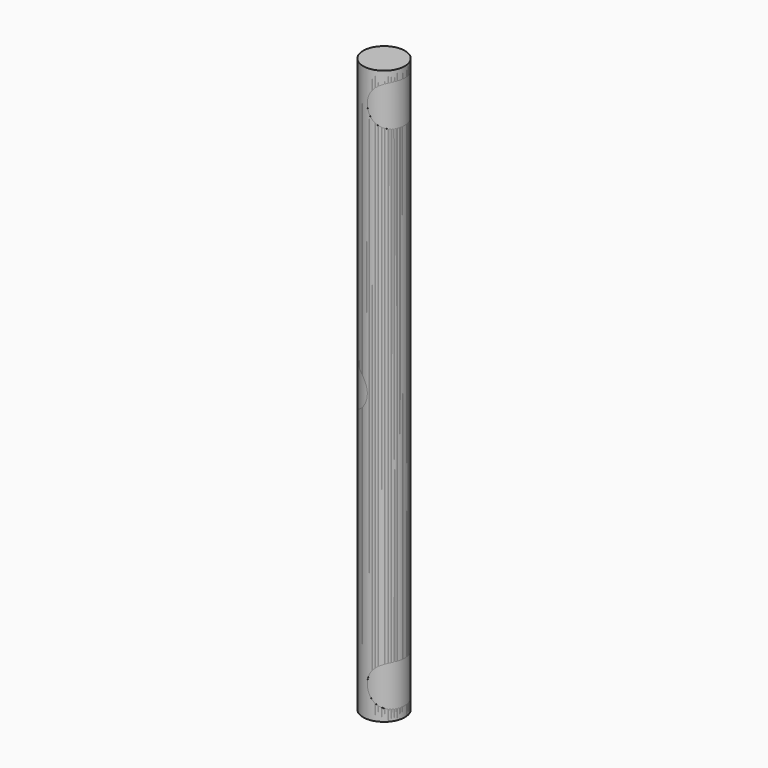
from build123d import *

# Parameters (mm, degrees)
F0_R     = 4
F1_DEPTH = 110
F2_R     = 4
F3_DEPTH = 110
F6_DEPTH = 25


with BuildPart() as f1:
    # F0 (on Top) → F1 (new body)
    with BuildSketch(Plane.XY):
        Circle(F0_R)
    extrude(amount=F1_DEPTH)


with BuildPart() as f3:
    # F2 (on Top) → F3 (new body)
    with BuildSketch(Plane.XY):
        Circle(F2_R)
    extrude(amount=F3_DEPTH)

    # F5 (on offset) → F6 (cut)
    with BuildSketch(Plane.XZ.offset(4)):
        with BuildLine():
            ThreePointArc((4, 108), (0, 104), (4, 100))
            Line((4, 100), (4, 108))
        make_face()
        with BuildLine():
            Line((-4, 59), (-4, 51))
            ThreePointArc((-4, 51), (0, 55), (-4, 59))
        make_face()
        with BuildLine():
            ThreePointArc((4, 10), (0, 6), (4, 2))
            Line((4, 2), (4, 10))
        make_face()
    extrude(amount=-F6_DEPTH, mode=Mode.SUBTRACT)


solid = Compound([f1.part, f3.part])
